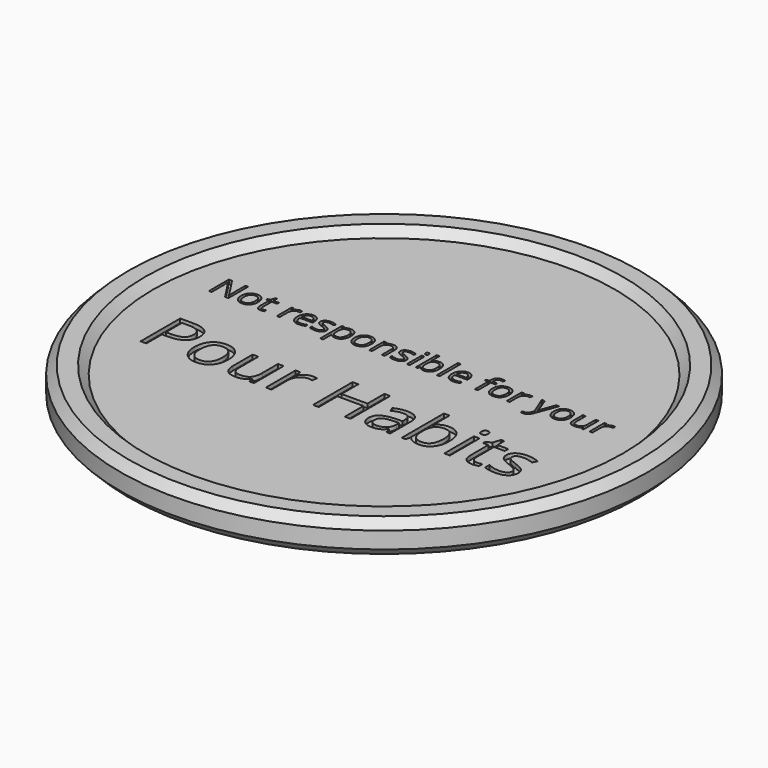
from build123d import *

# Parameters (mm, degrees)
F2_SIZE        = 1.58749
F3_TEXT_SIZE   = 6.6145833333
F3_TEXT_SIZE_2 = 13.2291666667
F4_DEPTH       = 0.79375


# Not quite as in the source:
# - a fillet or chamfer is up to 0.001 mm smaller than in the source, because OpenCascade refuses the exact size
# - Text() gives the source's letters only with a copy of the font that has no kerning and outlines rounded to 1/6400 em; it was checked with that copy


with BuildPart() as f1:
    # F0 (on Front) → F1 (revolve)
    with BuildSketch(Plane.XZ):
        Polygon((0, 4.7625), (0, 0), (50.403125, 0), (50.403125, 6.35), (45.640625, 6.35), (45.640625, 4.7625), align=None)
    revolve(axis=Axis((0, 0, 37.571658917), (0, 0, 1)))

    # F2 (size 1.5875 in the source; OpenCascade refuses exactly that, so slightly less here)
    f2_edges = [f1.edges().sort_by_distance(p)[0] for p in [
        (-45.640625, 0, 4.7625),
        (-50.403125, 0, 0),
        (-50.403125, 0, 6.35),
    ]]
    chamfer(f2_edges, length=F2_SIZE)

    # F3 (on face) → F4 (cut)
    with BuildSketch(Plane.XY.offset(4.7625)):
        with Locations((-37.8891601563, 4.7625)):
            Text('Not responsible for your', F3_TEXT_SIZE, font='Open Sans', text_align=(TextAlign.LEFT, TextAlign.BOTTOM))
        with Locations((-36.3574707031, -14.2875)):
            Text('Pour Habits', F3_TEXT_SIZE_2, font='Open Sans', text_align=(TextAlign.LEFT, TextAlign.BOTTOM))
    extrude(amount=-F4_DEPTH, mode=Mode.SUBTRACT)


solid = f1.part
